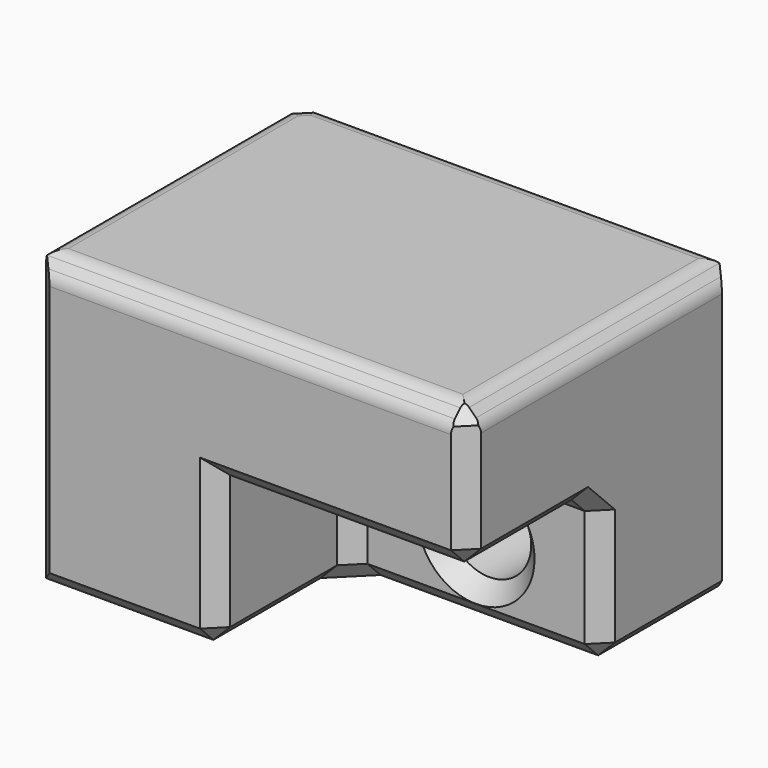
from build123d import *

# Parameters (mm, degrees)
F0_W         = 52
F0_H         = 35
F1_DEPTH     = 40
F2_W         = 30
F2_H         = 18
F3_DEPTH     = 20
F4_R         = 5
F5_DEPTH     = 20.001
F6_SIZE      = 1.99999
F7_T1_DEPTH  = 40.1421556237
F7_T3_DEPTH  = 42.1421456237
F7_T5_DEPTH  = 46.00002
F7_T7_DEPTH  = 12.8284129826
F7_T9_DEPTH  = 54.1421456237
F7_T11_DEPTH = 58.00002
F7_T13_DEPTH = 52.1421556237


# Not quite as in the source:
# - a fillet or chamfer that OpenCascade refuses, or shapes differently, is made with other operations: its cross-section is extruded or revolved along the edge and cut away or added
# - a fillet or chamfer is up to 0.001 mm smaller than in the source, because OpenCascade refuses the exact size


with BuildPart() as f1:
    # F0 (on Front) → F1 (new body)
    with BuildSketch(Plane.XZ):
        with Locations((16.8289473057, -27.5394749641)):
            Rectangle(F0_W, F0_H)
    extrude(amount=F1_DEPTH)

    # F2 (on face) → F3 (cut)
    with BuildSketch(Plane.XZ.offset(40)):
        with Locations((27.8289473057, -36.0394749641)):
            Rectangle(F2_W, F2_H)
    extrude(amount=-F3_DEPTH, mode=Mode.SUBTRACT)

    # F4 (on face) → F5 (cut, through all)
    with BuildSketch(Plane.XZ.offset(20)):
        with Locations((27.8289473057, -36.0394749641)):
            Circle(F4_R)
    extrude(amount=-F5_DEPTH, mode=Mode.SUBTRACT)

    # F6 (size 2 in the source; OpenCascade refuses exactly that, so slightly less here)
    f6_edges = [f1.edges().sort_by_distance(p)[0] for p in [
        (-9.171053, -40, -27.539475),
        (16.828947, -40, -10.039475),
        (42.828947, -40, -18.539475),
        (27.828947, -40, -27.039475),
        (12.828947, -40, -36.039475),
        (1.828947, -40, -45.039475),
        (-9.171053, 0, -27.539475),
        (27.828947, -20, -45.039475),
        (12.828947, -20, -36.039475),
        (42.828947, -20, -36.039475),
        (27.828947, -20, -27.039475),
        (22.828947, -20, -36.039475),
        (42.828947, 0, -27.539475),
        (42.828947, -20, -10.039475),
        (42.828947, -30, -27.039475),
        (42.828947, -10, -45.039475),
        (12.828947, -30, -45.039475),
    ]]
    chamfer(f6_edges, length=F6_SIZE)

    # F7: fillet of radius 2 on 7 edges, made by hand

    # F7_s2 → F7_t1 (cut)
    with BuildSketch(Plane.XZ.offset(-0.0710778119)):
        with BuildLine():
            ThreePointArc((42.8289473057, -12.8678920889), (42.6767063707, -12.1025252242), (42.2431608681, -11.4536785265))
            Line((42.2431608681, -11.4536785265), (42.8289473057, -12.0394649641))
            Line((42.8289473057, -12.0394649641), (42.8289473057, -12.8678920889))
        make_face()
    extrude(amount=F7_T1_DEPTH, mode=Mode.SUBTRACT)

    # F7_s4 → F7_t3 (cut)
    with BuildSketch(Plane.XZ.offset(-2.0710678119)):
        with BuildLine():
            ThreePointArc((40.0005301809, -10.0394749641), (40.7658970457, -10.1917158991), (41.4147437433, -10.6252614018))
            Line((41.4147437433, -10.6252614018), (40.8289573057, -10.0394749641))
            Line((40.8289573057, -10.0394749641), (40.0005301809, -10.0394749641))
        make_face()
    extrude(amount=F7_T3_DEPTH, mode=Mode.SUBTRACT)

    # F7_s6 → F7_t5 (cut)
    with BuildSketch(Plane.XZ.offset(-3.00001)):
        with BuildLine():
            ThreePointArc((-9.1710526943, -12.0394749641), (-8.5852662567, -10.6252614018), (-7.1710526943, -10.0394749641))
            Line((-7.1710526943, -10.0394749641), (-9.1710526943, -10.0394749641))
            Line((-9.1710526943, -10.0394749641), (-9.1710526943, -12.0394749641))
        make_face()
    extrude(amount=F7_T5_DEPTH, mode=Mode.SUBTRACT)

    # F7_s8 → F7_t7 (cut)
    with BuildSketch(Plane(origin=(-0.0499974412, -0.0499974412, 0), x_dir=(0, 0, 1), z_dir=(-0.7071067812, -0.7071067812, 0))):
        with BuildLine():
            ThreePointArc((-12.0394749641, 5.0707070595), (-10.6252614018, 4.4849206218), (-10.0394749641, 3.0707070595))
            Line((-10.0394749641, 3.0707070595), (-10.0394749641, 5.0707070595))
            Line((-10.0394749641, 5.0707070595), (-12.0394749641, 5.0707070595))
        make_face()
    extrude(amount=F7_T7_DEPTH, mode=Mode.SUBTRACT)

    # F7_s10 → F7_t9 (cut)
    with BuildSketch(Plane.YZ.offset(-11.2421205062)):
        with BuildLine():
            ThreePointArc((-37.1715828753, -10.0394749641), (-37.93694974, -10.1917158991), (-38.5857964376, -10.6252614018))
            Line((-38.5857964376, -10.6252614018), (-38.00001, -10.0394749641))
            Line((-38.00001, -10.0394749641), (-37.1715828753, -10.0394749641))
        make_face()
    extrude(amount=F7_T9_DEPTH, mode=Mode.SUBTRACT)

    # F7_s12 → F7_t11 (cut)
    with BuildSketch(Plane.YZ.offset(-12.1710626943)):
        with BuildLine():
            ThreePointArc((0, -12.0394749641), (-0.5857864376, -10.6252614018), (-2, -10.0394749641))
            Line((-2, -10.0394749641), (0, -10.0394749641))
            Line((0, -10.0394749641), (0, -12.0394749641))
        make_face()
    extrude(amount=F7_T11_DEPTH, mode=Mode.SUBTRACT)

    # F7_s14 → F7_t13 (cut)
    with BuildSketch(Plane.YZ.offset(-9.2421305062)):
        with BuildLine():
            ThreePointArc((-40, -12.8678920889), (-39.847759065, -12.1025252242), (-39.4142135624, -11.4536785265))
            Line((-39.4142135624, -11.4536785265), (-40, -12.0394649641))
            Line((-40, -12.0394649641), (-40, -12.8678920889))
        make_face()
    extrude(amount=F7_T13_DEPTH, mode=Mode.SUBTRACT)


solid = f1.part
